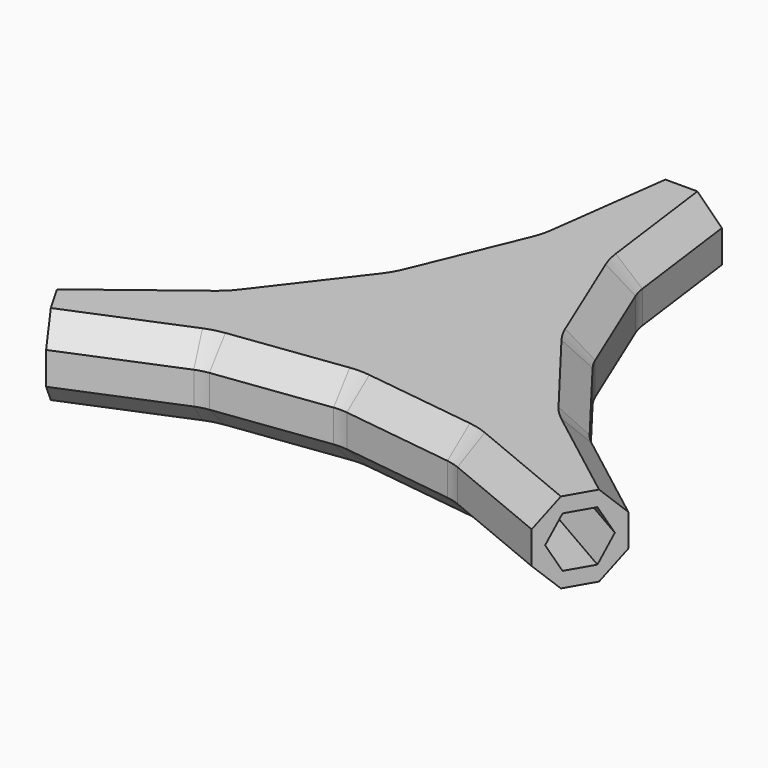
from build123d import *

# Parameters (mm, degrees)
F3_DEPTH        = 5.08
F4_R            = 6.35
F5_SIZE         = 3.048
F7_DEPTH        = 12.7
F7_COPIES_COUNT = 3


# Not quite as in the source:
# - a pattern or mirror of a feature is missing from the dataset's text; its kind, count and spacing are read off the source's solid


with BuildPart() as f3:
    # F2 (on Top) → F3 (new body, symmetric)
    with BuildSketch(Plane.XY):
        Polygon((7.1554966211, 22.3350380043), (5.08, 38.1), (-5.08, 38.1), (-7.1554966211, 22.3350380043), (-13.2405448196, 7.6444321158), (-22.9204586168, -4.9706771516), (-35.5355678842, -14.6505909488), (-30.4555678842, -23.4494090512), (-15.7649619957, -17.3643608527), (0, -15.2888642316), (15.7649619957, -17.3643608527), (30.4555678842, -23.4494090512), (35.5355678842, -14.6505909488), (22.9204586168, -4.9706771516), (13.2405448196, 7.6444321158), align=None)
    extrude(amount=F3_DEPTH, both=True)

    # F4
    f4_edges = [f3.edges().sort_by_distance(p)[0] for p in [
        (-22.920459, -4.970677, 0),
        (-13.240545, 7.644432, 0),
        (7.155497, 22.335038, 0),
        (13.240545, 7.644432, 0),
        (-15.764962, -17.364361, 0),
        (0, -15.288864, 0),
        (22.920459, -4.970677, 0),
        (-7.155497, 22.335038, 0),
        (15.764962, -17.364361, 0),
    ]]
    fillet(f4_edges, radius=F4_R)

    # F5
    f5_edges = [f3.edges().sort_by_distance(p)[0] for p in [
        (-23.496444, -20.566845, 5.08),
        (-7.882481, -16.326613, 5.08),
        (7.882481, -16.326613, 5.08),
        (-29.559632, -10.065094, 5.08),
        (-18.080502, 1.336877, 5.08),
        (-10.198021, 14.989735, 5.08),
        (6.063189, 30.63194, 5.08),
        (10.198021, 14.989735, 5.08),
        (18.080502, 1.336877, 5.08),
        (-29.559632, -10.065094, -5.08),
        (-18.080502, 1.336877, -5.08),
        (-10.198021, 14.989735, -5.08),
        (6.063189, 30.63194, -5.08),
        (10.198021, 14.989735, -5.08),
        (18.080502, 1.336877, -5.08),
        (7.882481, -16.326613, -5.08),
        (-7.882481, -16.326613, -5.08),
        (-23.496444, -20.566845, -5.08),
        (-15.75078, -17.417288, -5.08),
        (0, -15.343658, -5.08),
        (15.75078, -17.417288, -5.08),
        (23.496444, -20.566845, -5.08),
        (-22.959204, -4.931932, -5.08),
        (29.559632, -10.065094, -5.08),
        (-13.287998, 7.671829, -5.08),
        (22.959204, -4.931932, -5.08),
        (-7.208423, 22.34922, -5.08),
        (13.287998, 7.671829, -5.08),
        (-6.063189, 30.63194, -5.08),
        (7.208423, 22.34922, -5.08),
        (-15.75078, -17.417288, 5.08),
        (0, -15.343658, 5.08),
        (15.75078, -17.417288, 5.08),
        (23.496444, -20.566845, 5.08),
        (-22.959204, -4.931932, 5.08),
        (29.559632, -10.065094, 5.08),
        (-13.287998, 7.671829, 5.08),
        (22.959204, -4.931932, 5.08),
        (-7.208423, 22.34922, 5.08),
        (13.287998, 7.671829, 5.08),
        (-6.063189, 30.63194, 5.08),
        (7.208423, 22.34922, 5.08),
    ]]
    chamfer(f5_edges, length=F5_SIZE)

    # F6 (on face) → F7 (cut)
    with BuildSketch(Plane(origin=(32.9955678842, -19.05, 0), x_dir=(0.5, 0.8660254038, 0), z_dir=(0.8660254038, -0.5, 0))):
        Polygon((-1.8330871047, 3.175), (-3.6661742094, 0), (-1.8330871047, -3.175), (1.8330871047, -3.175), (3.6661742094, 0), (1.8330871047, 3.175), align=None)
    f7 = extrude(amount=-F7_DEPTH, mode=Mode.SUBTRACT)

    # F7_copies: F7 ×3 about axis
    f7_copies_axis = Axis((0, 0, 0), (0, 0, 1))
    for i in range(1, F7_COPIES_COUNT):
        add(f7.rotate(f7_copies_axis, i * 360 / F7_COPIES_COUNT), mode=Mode.SUBTRACT)


solid = f3.part
